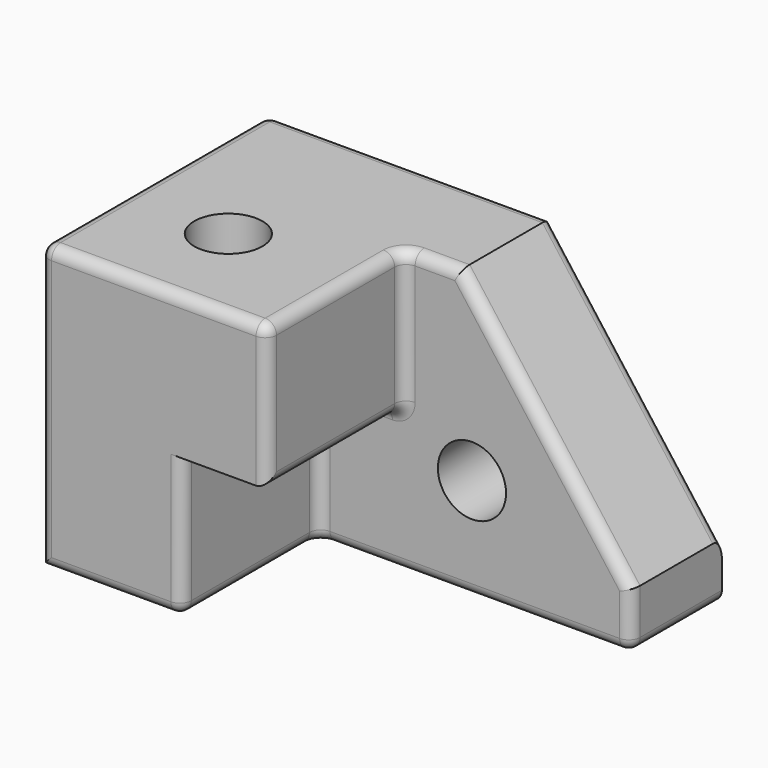
from build123d import *

# Parameters (mm, degrees)
F0_W     = 203.2
F0_H     = 127
F1_DEPTH = 127
F3_DEPTH = 76.2
F4_SIZE2 = 101.6
F4_SIZE  = 76.2
F5_R     = 5.08
F6_R     = 15.24
F7_DEPTH = 50.8
F8_R     = 15.24
F9_DEPTH = 127


with BuildPart() as f1:
    # F0 (on Front) → F1 (new body)
    with BuildSketch(Plane.XZ):
        with Locations((-1.3009174736, 0.3703823313)):
            Rectangle(F0_W, F0_H)
    extrude(amount=F1_DEPTH)

    # F2 (on face) → F3 (cut)
    with BuildSketch(Plane.XZ.offset(127)):
        Polygon((-39.4009174736, 0), (-39.4009174736, -63.1296176687), (100.2990825264, -63.1296176687), (100.2990825264, 63.8703823313), (-1.3009174736, 63.8703823313), (-1.3009174736, 0), align=None)
    extrude(amount=-F3_DEPTH, mode=Mode.SUBTRACT)

    # F4
    f4_edges = [f1.edges().sort_by_distance(p)[0] for p in [
        (100.299083, -25.4, 63.870382),
    ]]
    f4_side = f1.faces().sort_by_distance((-23.072346, -52.614286, 63.870382))[0]
    chamfer(f4_edges, length=F4_SIZE, length2=F4_SIZE2, reference=f4_side)

    # F5
    f5_edges = [f1.edges().sort_by_distance(p)[0] for p in [
        (11.399083, -50.8, 63.870382),
        (-1.300917, -88.9, 63.870382),
        (-52.100917, -127, 63.870382),
        (100.299083, -50.8, -50.429618),
        (62.199083, -50.8, 13.070382),
        (30.449083, -50.8, -63.129618),
        (-39.400917, -50.8, -31.564809),
        (-1.300917, -50.8, 31.935191),
        (-20.350917, -50.8, 0),
        (-1.300917, -127, 31.935191),
        (-1.300917, -88.9, 0),
        (-39.400917, -127, -31.564809),
        (100.299083, -25.4, -63.129618),
        (-71.150917, -127, -63.129618),
        (-39.400917, 0, 63.870382),
        (62.199083, 0, 13.070382),
        (-102.900917, -63.5, 63.870382),
        (-102.900917, -127, 0.370382),
        (-102.900917, 0, 0.370382),
        (-39.400917, -88.9, -63.129618),
    ]]
    fillet(f5_edges, radius=F5_R)

    # F6 (on face) → F7 (cut, through all)
    with BuildSketch(Plane.XZ.offset(50.8)):
        with Locations((29.1790825264, -17.4096176687)):
            Circle(F6_R)
    extrude(amount=-F7_DEPTH, mode=Mode.SUBTRACT)

    # F8 (on face) → F9 (cut, through all)
    with BuildSketch(Plane.XY.offset(63.8703823313)):
        with Locations((-56.2786398957, -80.1086086328)):
            Circle(F8_R)
    extrude(amount=-F9_DEPTH, mode=Mode.SUBTRACT)


solid = f1.part
